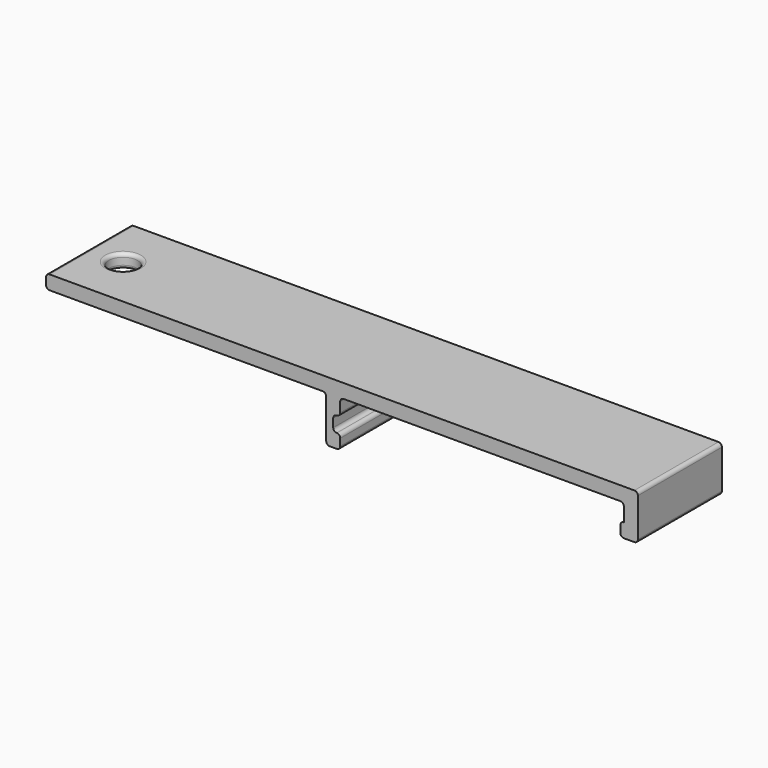
from build123d import *

# Parameters (mm, degrees)
F1_DEPTH = 15
F2_R     = 2.05
F3_DEPTH = 25
F4_R     = 0.49999


# Not quite as in the source:
# - a fillet or chamfer is up to 0.001 mm smaller than in the source, because OpenCascade refuses the exact size


with BuildPart() as f1:
    # F0 (on Front) → F1 (new body)
    with BuildSketch(Plane.XZ):
        Polygon((-0.25, -2), (-2.25, -2), (-2.25, -8.6), (-0.25, -8.6), (-0.25, -6.6), (-1.25, -6.6), (-1.25, -4.4), (-0.25, -4.4), align=None)
        Polygon((42.25, 0), (-42.25, 0), (-42.25, -2), (-2.25, -2), (-0.25, -2), (40.25, -2), (42.25, -2), align=None)
        Polygon((42.25, -6.5), (42.25, -2), (40.25, -2), (40.25, -4.5), (39.75, -4.5), (39.75, -6.5), align=None)
    extrude(amount=F1_DEPTH)

    # F2 (on face) → F3 (cut)
    with BuildSketch(Plane.XY):
        with Locations((-37.25, -7.5)):
            Circle(F2_R)
    extrude(amount=-F3_DEPTH, mode=Mode.SUBTRACT)

    # F4 (radius 0.5 in the source; OpenCascade refuses exactly that, so slightly less here)
    f4_edges = [f1.edges().sort_by_distance(p)[0] for p in [
        (-1.25, -7.5, -6.6),
        (-0.25, -7.5, -8.6),
        (39.75, -7.5, -6.5),
        (39.75, -7.5, -4.5),
        (-39.3, -7.5, 0),
        (42.25, -7.5, 0),
        (42.25, -7.5, -6.5),
        (-42.25, -7.5, 0),
        (-42.25, -7.5, -2),
        (-2.25, -7.5, -2),
        (-0.25, -7.5, -2),
        (40.25, -7.5, -2),
        (-2.25, -7.5, -8.6),
        (-39.3, -7.5, -2),
        (-0.25, -7.5, -4.4),
        (-1.25, -7.5, -4.4),
        (-0.25, -7.5, -6.6),
    ]]
    fillet(f4_edges, radius=F4_R)


solid = f1.part
